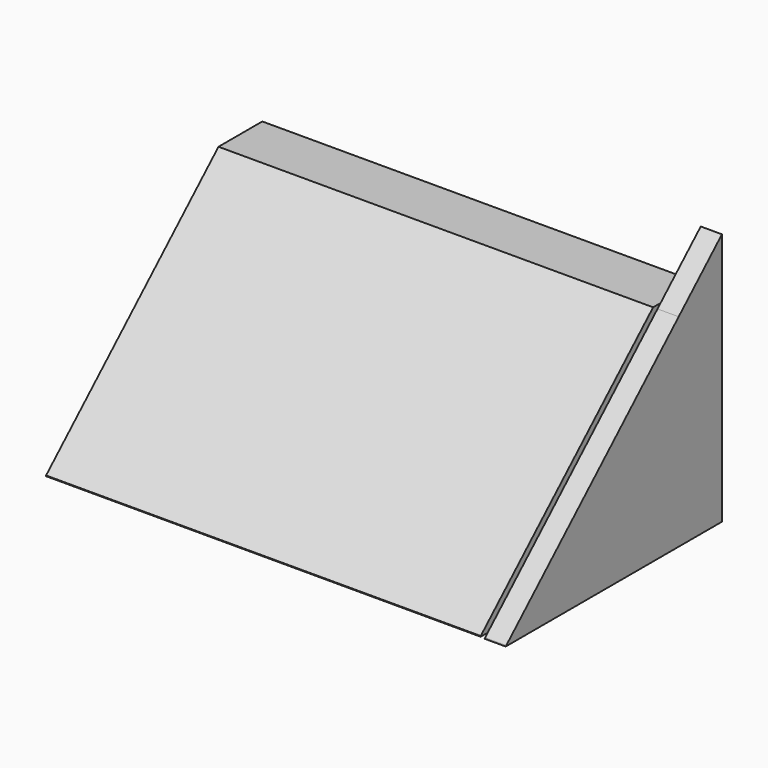
from build123d import *

# Parameters (mm, degrees)
F0_W     = 109.0628877282
F0_H     = 67.8206197917
F1_DEPTH = 50.8
F2_W     = 5.3156651556
F2_H     = 67.8206197917
F3_DEPTH = 63.5
F5_DEPTH = 127


# Not quite as in the source:
# - a feature of the source that left no trace in its solid (it failed there, or was rolled back) is left out


with BuildPart() as f1:
    # F0 (on Top) → F1 (new body)
    with BuildSketch(Plane.XY):
        with Locations((-1.0081455112, 0.6415452808)):
            Rectangle(F0_W, F0_H)
    extrude(amount=F1_DEPTH)


with BuildPart() as f3:
    # F2 (on Top) → F3 (new body)
    with BuildSketch(Plane.XY):
        with Locations((57.2809297591, 0.458246097)):
            Rectangle(F2_W, F2_H)
    extrude(amount=F3_DEPTH)


with BuildPart() as f5_tool:
    # F4 (on face) → F5 (new body)
    with BuildSketch(Plane(origin=(-55.5395893753, 0, 0), x_dir=(0, -1, 0), z_dir=(-1, 0, 0))):
        Polygon((-34.3685559928, 63.5), (-20.8044320345, 50.8), (33.2687646151, 50.8), (33.2687646151, 0.1716218196), (33.4520637989, 0), (33.4520637989, 63.5), align=None)
        Polygon((33.2687646151, 50.8), (-20.8044320345, 50.8), (33.2687646151, 0.1716218196), align=None)
    extrude(amount=-F5_DEPTH)


with BuildPart() as f1_1:
    add(f1.part)

    # F5: cut by f5_tool
    add(f5_tool.part, mode=Mode.SUBTRACT)


with BuildPart() as f3_1:
    add(f3.part)

    # F5: cut by f5_tool
    add(f5_tool.part, mode=Mode.SUBTRACT)


solid = Compound([f1_1.part, f3_1.part])
